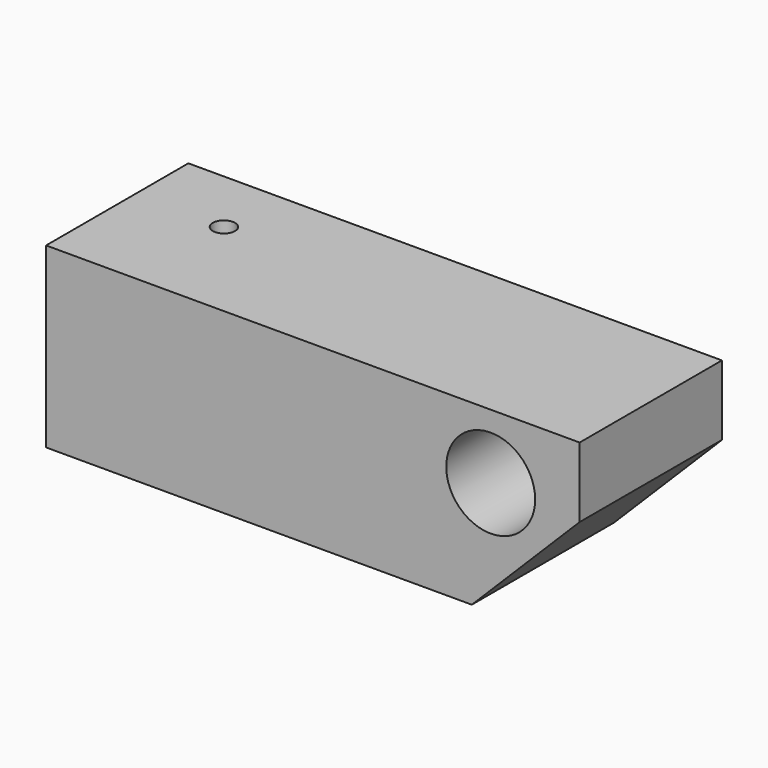
from build123d import *

# Parameters (mm, degrees)
F1_DEPTH = 50.8
F2_W     = 12.7
F2_H     = 38.1
F3_DEPTH = 50.8
F5_D     = 25.4
F7_D     = 6.35


# Not quite as in the source:
# - a feature names something its author has since deleted; it is built from what else it names


with BuildPart() as f1:
    # F0 (on Front) → F1 (new body)
    with BuildSketch(Plane.XZ):
        Polygon((-140.8084735786, 36.6746302678), (-140.8084735786, 30.3246302678), (-90.0084735786, 30.3246302678), (-90.0084735786, -7.7753697322), (-140.8084735786, -7.7753697322), (-140.8084735786, -14.1253697322), (-19.2084735786, -14.1253697322), (11.5915264214, 16.6746302678), (11.5915264214, 36.6746302678), align=None)
    extrude(amount=F1_DEPTH)

    # F2 (on face) → F3 (join)
    with BuildSketch(Plane(origin=(-90.0084735786, 0, 0), x_dir=(0, -1, 0), z_dir=(-1, 0, 0))):
        with Locations((44.45, 11.2746302678)):
            Rectangle(F2_W, F2_H)
    extrude(amount=F3_DEPTH)

    # F5 (through all)
    with Locations(Plane(origin=(0, 0, 0), x_dir=(-1, 0, 0), z_dir=(0, 1, 0))):
        with Locations((13.8084735786, 18.215398631)):
            Hole(F5_D / 2)

    # F7 (through all)
    with Locations(Plane.XY.offset(36.6746302678)):
        with Locations((-115.4084735786, -19.05)):
            Hole(F7_D / 2)


solid = f1.part
